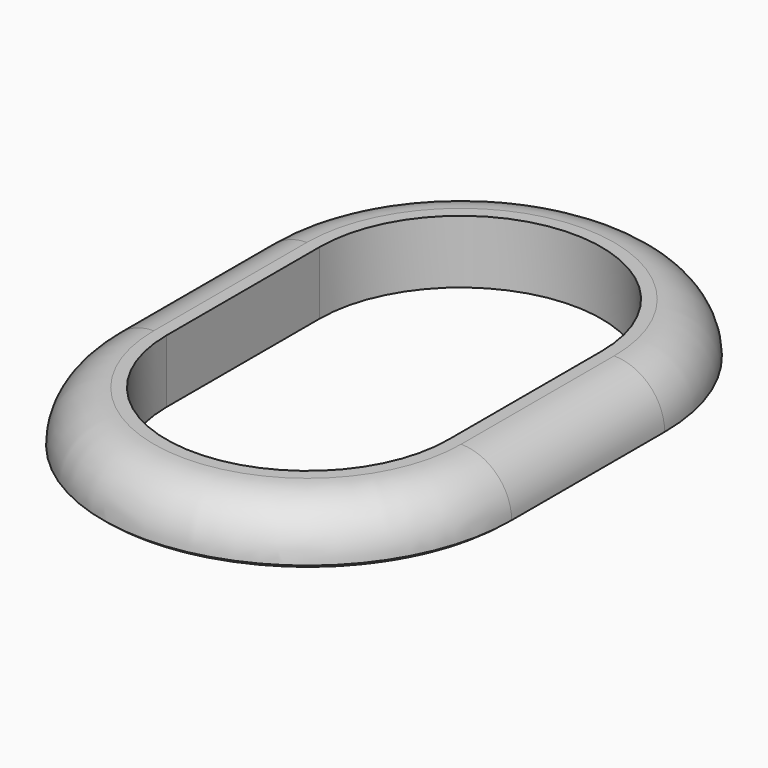
from build123d import *

# Parameters (mm, degrees)
F1_DEPTH    = 6.35
F2_R        = 5.08
F3_T1_DEPTH = 19.2442405969
F3_T4_ANGLE = 180
F3_T6_ANGLE = 180


# Not quite as in the source:
# - a fillet or chamfer that OpenCascade refuses, or shapes differently, is made with other operations: its cross-section is extruded or revolved along the edge and cut away or added


with BuildPart() as f1:
    # F0 (on Top) → F1 (new body)
    with BuildSketch(Plane.XY):
        with BuildLine():
            Line((20.5361241051, 0), (20.5361241051, 19.2442405969))
            ThreePointArc((20.5361241051, 19.2442405969), (0, 39.780364702), (-20.5361241051, 19.2442405969))
            Line((-20.5361241051, 19.2442405969), (-20.5361241051, 0))
            ThreePointArc((-20.5361241051, 0), (0, -20.5361241051), (20.5361241051, 0))
        make_face()
        with BuildLine():
            ThreePointArc((14.1861241051, 0), (0, -14.1861241051), (-14.1861241051, 0))
            Line((-14.1861241051, 0), (-14.1861241051, 19.2442405969))
            ThreePointArc((-14.1861241051, 19.2442405969), (0, 33.430364702), (14.1861241051, 19.2442405969))
            Line((14.1861241051, 19.2442405969), (14.1861241051, 0))
        make_face(mode=Mode.SUBTRACT)
    extrude(amount=F1_DEPTH)

    # F2
    f2_edges = [f1.edges().sort_by_distance(p)[0] for p in [
        (0, 39.780365, 6.35),
    ]]
    fillet(f2_edges, radius=F2_R)

    # F3: fillet of radius 5.08 on 1 edges, made by hand

    # F3_s2 → F3_t1 (cut)
    with BuildSketch(Plane.XZ.offset(-19.2442405969)):
        with BuildLine():
            ThreePointArc((20.5361241051, 1.27), (18.9720711643, 0.3280951188), (17.1760199401, 0))
            Line((17.1760199401, 0), (20.5361241051, 0))
            Line((20.5361241051, 0), (20.5361241051, 1.27))
        make_face()
        with BuildLine():
            ThreePointArc((-17.1760199401, 0), (-18.9720711643, 0.3280951188), (-20.5361241051, 1.27))
            Line((-20.5361241051, 1.27), (-20.5361241051, 0))
            Line((-20.5361241051, 0), (-17.1760199401, 0))
        make_face()
    extrude(amount=F3_T1_DEPTH, mode=Mode.SUBTRACT)

    # F3_s3 → F3_t4 (revolve, cut)
    with BuildSketch(Plane.XZ.offset(-19.2442405969)):
        with BuildLine():
            ThreePointArc((17.1760199401, 0), (18.9720711643, 0.3280951188), (20.5361241051, 1.27))
            Line((20.5361241051, 1.27), (20.5361241051, 0))
            Line((20.5361241051, 0), (17.1760199401, 0))
        make_face()
    revolve(axis=Axis((0, 19.2442405969, 0), (0, 0, 1)), revolution_arc=F3_T4_ANGLE, mode=Mode.SUBTRACT)

    # F3_s5 → F3_t6 (revolve, cut)
    with BuildSketch(Plane.XZ):
        with BuildLine():
            ThreePointArc((-20.5361241051, 1.27), (-18.9720711643, 0.3280951188), (-17.1760199401, 0))
            Line((-17.1760199401, 0), (-20.5361241051, 0))
            Line((-20.5361241051, 0), (-20.5361241051, 1.27))
        make_face()
    revolve(axis=Axis((0, 0, 0), (0, 0, 1)), revolution_arc=F3_T6_ANGLE, mode=Mode.SUBTRACT)


solid = f1.part
